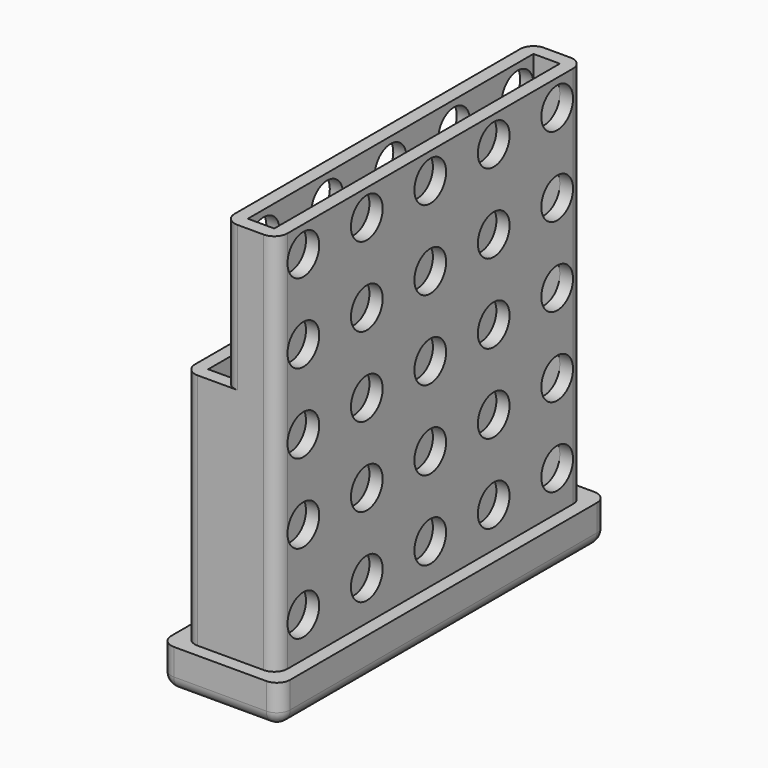
from build123d import *

# Parameters (mm, degrees)
F0_W     = 4
F0_H     = 54
F1_DEPTH = 62
F2_DEPTH = 40
F4_R     = 2
F5_R     = 3
F6_DEPTH = 14.001
F8_DEPTH = 2
F9_DEPTH = 4
F10_R    = 1.99999


# Not quite as in the source:
# - a fillet or chamfer is up to 0.001 mm smaller than in the source, because OpenCascade refuses the exact size
# - a feature of the source that left no trace in its solid (it failed there, or was rolled back) is left out


with BuildPart() as f1:
    # F0 (on Top) → F1 (new body)
    with BuildSketch(Plane.XY):
        Polygon((4, -29), (4, 29), (-4, 29), (-4, 27), (-4, -27), (-4, -29), align=None)
        Rectangle(F0_W, F0_H, mode=Mode.SUBTRACT)
    extrude(amount=F1_DEPTH)

    # F0 (on Top) → F2 (join)
    with BuildSketch(Plane.XY):
        Polygon((-4, 27), (-4, 29), (-10, 29), (-10, 27), (-10, -27), (-10, -29), (-4, -29), (-4, -27), (-8, -27), (-8, 27), align=None)
    extrude(amount=F2_DEPTH)

    # F4
    f4_edges = [f1.edges().sort_by_distance(p)[0] for p in [
        (4, -29, 31),
        (4, 29, 31),
    ]]
    fillet(f4_edges, radius=F4_R)

    # F5 (on face) → F6 (cut, through all)
    with BuildSketch(Plane.YZ.offset(4)):
        with Locations((-24, 10)):
            Circle(F5_R)
        with Locations((-24, 22)):
            Circle(F5_R)
        with Locations((-24, 34)):
            Circle(F5_R)
        with Locations((-24, 46)):
            Circle(F5_R)
        with Locations((-12, 10)):
            Circle(F5_R)
        with Locations((-12, 22)):
            Circle(F5_R)
        with Locations((-12, 34)):
            Circle(F5_R)
        with Locations((-12, 46)):
            Circle(F5_R)
        with Locations((0, 10)):
            Circle(F5_R)
        with Locations((0, 22)):
            Circle(F5_R)
        with Locations((0, 34)):
            Circle(F5_R)
        with Locations((0, 46)):
            Circle(F5_R)
        with Locations((12, 10)):
            Circle(F5_R)
        with Locations((12, 22)):
            Circle(F5_R)
        with Locations((12, 34)):
            Circle(F5_R)
        with Locations((12, 46)):
            Circle(F5_R)
        with Locations((24, 10)):
            Circle(F5_R)
        with Locations((24, 22)):
            Circle(F5_R)
        with Locations((24, 34)):
            Circle(F5_R)
        with Locations((24, 46)):
            Circle(F5_R)
        with Locations((-24, 58)):
            Circle(F5_R)
        with Locations((-12, 58)):
            Circle(F5_R)
        with Locations((0, 58)):
            Circle(F5_R)
        with Locations((12, 58)):
            Circle(F5_R)
        with Locations((24, 58)):
            Circle(F5_R)
    extrude(amount=-F6_DEPTH, mode=Mode.SUBTRACT)

    # F7 (on face) → F8 (join)
    with BuildSketch(Plane.XY):
        with BuildLine():
            ThreePointArc((4, -31), (5.4142135624, -30.4142135624), (6, -29))
            Line((6, -29), (6, 29))
            ThreePointArc((6, 29), (5.4142135624, 30.4142135624), (4, 31))
            Line((4, 31), (-10, 31))
            ThreePointArc((-10, 31), (-11.4142135624, 30.4142135624), (-12, 29))
            Line((-12, 29), (-12, -29))
            ThreePointArc((-12, -29), (-11.4142135624, -30.4142135624), (-10, -31))
            Line((-10, -31), (4, -31))
        make_face()
    extrude(amount=-F8_DEPTH)

    # F9 (add): a face of the model
    f9_faces = [f1.faces().sort_by_distance(p)[0] for p in [
        (-10.957705074, -29.957705074, 0),
    ]]
    extrude(f9_faces, amount=F9_DEPTH)

    # F10 (radius 2 in the source; OpenCascade refuses exactly that, so slightly less here)
    f10_edges = [f1.edges().sort_by_distance(p)[0] for p in [
        (6, 0, -2),
        (-11.414214, -30.414214, -2),
        (-12, 0, -2),
        (-11.414214, 30.414214, -2),
        (-3, 31, -2),
        (5.414214, 30.414214, -2),
        (5.414214, -30.414214, -2),
        (-4, -29, 51),
        (-4, 29, 51),
        (-10, -29, 22),
        (-10, 29, 22),
        (-3, -31, -2),
    ]]
    fillet(f10_edges, radius=F10_R)


solid = f1.part
